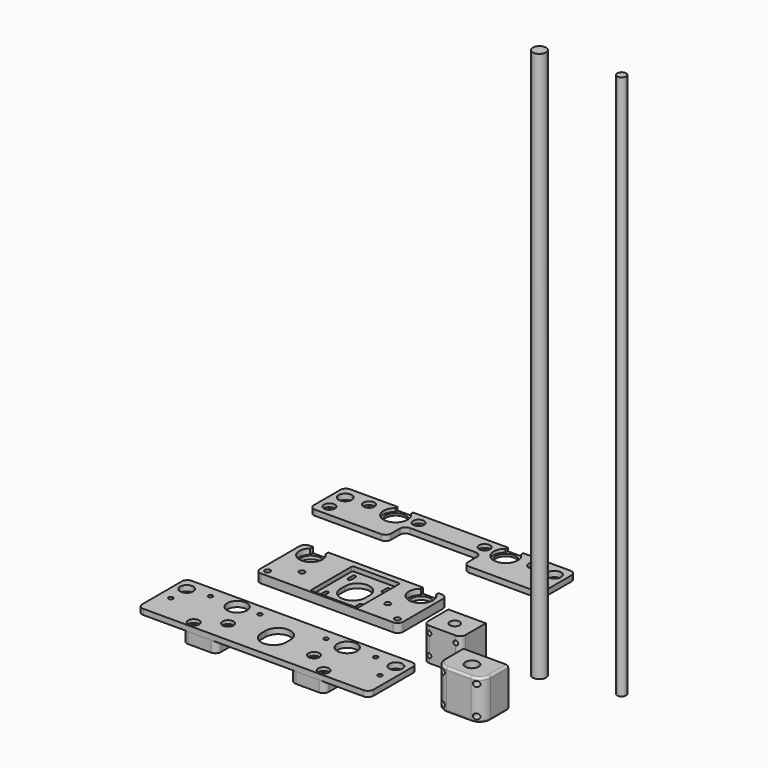
from build123d import *

# Parameters (mm, degrees)
F0_R         = 6
F1_DEPTH     = 500
F2_W         = 130
F2_H         = 55
F2_R         = 2.5
F2_W_2       = 43
F2_H_2       = 48
F2_R_2       = 9
F3_DEPTH     = 8
F4_DEPTH     = 4
F5_R         = 1
F6_R         = 9
F7_DEPTH     = 5
F8_R         = 5
F9_W         = 210
F9_H         = 55
F9_R         = 2.5
F9_R_2       = 2
F9_R_3       = 6
F9_R_4       = 9
F10_DEPTH    = 5
F11_R        = 5
F11_R_2      = 2.5
F12_DEPTH    = 3
F13_R        = 5
F14_W        = 31
F14_H        = 25
F14_R        = 2.5
F15_DEPTH    = 10
F16_R        = 5
F16_2_R      = 5
F17_R        = 2
F17_R_2      = 6
F17_R_3      = 9
F18_DEPTH    = 5
F19_R        = 9
F19_R_2      = 5
F19_R_3      = 2
F20_DEPTH    = 3
F21_R        = 5
F22_W        = 42
F22_H        = 30
F22_R        = 6
F23_DEPTH    = 36
F24_R        = 10
F25_R        = 2
F26_R        = 2.5
F27_DEPTH    = 40
F28_R        = 4
F29_DEPTH    = 495
F30_W        = 34
F30_H        = 28
F30_R        = 4.5
F31_DEPTH    = 30
F32_R        = 2
F33_DEPTH    = 35
F34_T1_DEPTH = 55


# Not quite as in the source:
# - a fillet or chamfer that OpenCascade refuses, or shapes differently, is made with other operations: its cross-section is extruded or revolved along the edge and cut away or added
# - a feature names something its author has since deleted; it is built from what else it names


with BuildPart() as f1:
    # F0 (on Top) → F1 (new body)
    with BuildSketch(Plane.XY):
        with Locations((45.0636185706, 37.0731987059)):
            Circle(F0_R)
    extrude(amount=F1_DEPTH)


with BuildPart() as f3:
    # F2 (on Top) → F3 (new body)
    with BuildSketch(Plane.XY):
        with Locations((-137.1023366213, 51.400513723)):
            Rectangle(F2_W, F2_H)
        with Locations((-196.1023366213, 29.900513723)):
            Circle(F2_R, mode=Mode.SUBTRACT)
        with Locations((-176.1023366213, 43.900513723)):
            Circle(F2_R, mode=Mode.SUBTRACT)
        with Locations((-78.1023366213, 29.900513723)):
            Circle(F2_R, mode=Mode.SUBTRACT)
        with Locations((-132.1023366213, 49.400513723)):
            Rectangle(F2_W_2, F2_H_2, mode=Mode.SUBTRACT)
        with Locations((-98.1023366213, 43.900513723)):
            Circle(F2_R, mode=Mode.SUBTRACT)
        with Locations((-187.1023366213, 67.900513723)):
            Circle(F2_R_2, mode=Mode.SUBTRACT)
        with Locations((-87.1023366213, 67.900513723)):
            Circle(F2_R_2, mode=Mode.SUBTRACT)
    extrude(amount=F3_DEPTH)

    # F2 (on Top) → F4 (join)
    with BuildSketch(Plane.XY):
        with Locations((-132.1023366213, 49.400513723)):
            Rectangle(F2_W_2, F2_H_2)
        with BuildLine():
            Line((-149.1523366213, 31.400513723), (-149.1523366213, 36.400513723))
            ThreePointArc((-149.1523366213, 36.400513723), (-147.6023366213, 37.950513723), (-146.0523366213, 36.400513723))
            Line((-146.0523366213, 36.400513723), (-146.0523366213, 31.400513723))
            ThreePointArc((-146.0523366213, 31.400513723), (-147.6023366213, 29.850513723), (-149.1523366213, 31.400513723))
        make_face(mode=Mode.SUBTRACT)
        with BuildLine():
            Line((-118.1523366213, 31.400513723), (-118.1523366213, 36.400513723))
            ThreePointArc((-118.1523366213, 36.400513723), (-116.6023366213, 37.950513723), (-115.0523366213, 36.400513723))
            Line((-115.0523366213, 36.400513723), (-115.0523366213, 31.400513723))
            ThreePointArc((-115.0523366213, 31.400513723), (-116.6023366213, 29.850513723), (-118.1523366213, 31.400513723))
        make_face(mode=Mode.SUBTRACT)
        with BuildLine():
            Line((-143.3523366213, 46.900513723), (-143.3523366213, 51.900513723))
            ThreePointArc((-143.3523366213, 51.900513723), (-132.1023366213, 63.150513723), (-120.8523366213, 51.900513723))
            Line((-120.8523366213, 51.900513723), (-120.8523366213, 46.900513723))
            ThreePointArc((-120.8523366213, 46.900513723), (-132.1023366213, 35.650513723), (-143.3523366213, 46.900513723))
        make_face(mode=Mode.SUBTRACT)
        with BuildLine():
            Line((-149.1523366213, 62.400513723), (-149.1523366213, 67.400513723))
            ThreePointArc((-149.1523366213, 67.400513723), (-147.6023366213, 68.950513723), (-146.0523366213, 67.400513723))
            Line((-146.0523366213, 67.400513723), (-146.0523366213, 62.400513723))
            ThreePointArc((-146.0523366213, 62.400513723), (-147.6023366213, 60.850513723), (-149.1523366213, 62.400513723))
        make_face(mode=Mode.SUBTRACT)
        with BuildLine():
            Line((-118.1523366213, 62.400513723), (-118.1523366213, 67.400513723))
            ThreePointArc((-118.1523366213, 67.400513723), (-116.6023366213, 68.950513723), (-115.0523366213, 67.400513723))
            Line((-115.0523366213, 67.400513723), (-115.0523366213, 62.400513723))
            ThreePointArc((-115.0523366213, 62.400513723), (-116.6023366213, 60.850513723), (-118.1523366213, 62.400513723))
        make_face(mode=Mode.SUBTRACT)
    extrude(amount=F4_DEPTH)

    # F5
    f5_edges = [f3.edges().sort_by_distance(p)[0] for p in [
        (-153.602337, 73.400514, 6),
        (-110.602337, 73.400514, 6),
        (-110.602337, 25.400514, 6),
        (-153.602337, 25.400514, 6),
    ]]
    fillet(f5_edges, radius=F5_R)

    # F6 (on face) → F7 (cut)
    with BuildSketch(Plane.XY.offset(8)):
        with BuildLine():
            ThreePointArc((-194.1023366213, 75.7267516443), (-191.3889436712, 58.3153689667), (-176.6023366213, 67.900513723))
            ThreePointArc((-176.6023366213, 67.900513723), (-177.5171918649, 72.1871207729), (-180.1023366213, 75.7267516443))
            ThreePointArc((-180.1023366213, 75.7267516443), (-187.1023366213, 78.400513723), (-194.1023366213, 75.7267516443))
        make_face()
        with Locations((-187.1023366213, 67.900513723)):
            Circle(F6_R, mode=Mode.SUBTRACT)
        with BuildLine():
            ThreePointArc((-194.1023366213, 75.7267516443), (-187.1023366213, 78.400513723), (-180.1023366213, 75.7267516443))
            Line((-180.1023366213, 75.7267516443), (-180.1023366213, 78.900513723))
            Line((-180.1023366213, 78.900513723), (-194.1023366213, 78.900513723))
            Line((-194.1023366213, 78.900513723), (-194.1023366213, 75.7267516443))
        make_face()
        with BuildLine():
            ThreePointArc((-87.1023366213, 78.900513723), (-90.8213354707, 78.2527621531), (-94.1023366213, 76.3857950973))
            ThreePointArc((-94.1023366213, 76.3857950973), (-91.7927523811, 57.950639352), (-76.1023366213, 67.900513723))
            ThreePointArc((-76.1023366213, 67.900513723), (-77.1524622502, 72.5909294829), (-80.1023366213, 76.3857950973))
            ThreePointArc((-80.1023366213, 76.3857950973), (-83.3833377719, 78.2527621531), (-87.1023366213, 78.900513723))
        make_face()
        with Locations((-87.1023366213, 67.900513723)):
            Circle(F6_R, mode=Mode.SUBTRACT)
        with BuildLine():
            Line((-87.1023366213, 78.900513723), (-94.1023366213, 78.900513723))
            Line((-94.1023366213, 78.900513723), (-94.1023366213, 76.3857950973))
            ThreePointArc((-94.1023366213, 76.3857950973), (-90.8213354707, 78.2527621531), (-87.1023366213, 78.900513723))
        make_face()
        with BuildLine():
            Line((-80.1023366213, 78.900513723), (-87.1023366213, 78.900513723))
            ThreePointArc((-87.1023366213, 78.900513723), (-83.3833377719, 78.2527621531), (-80.1023366213, 76.3857950973))
            Line((-80.1023366213, 76.3857950973), (-80.1023366213, 78.900513723))
        make_face()
    extrude(amount=-F7_DEPTH, mode=Mode.SUBTRACT)

    # F8
    f8_edges = [f3.edges().sort_by_distance(p)[0] for p in [
        (-202.102337, 78.900514, 4),
        (-202.102337, 23.900514, 4),
        (-72.102337, 23.900514, 4),
        (-72.102337, 78.900514, 4),
    ]]
    fillet(f8_edges, radius=F8_R)


with BuildPart() as f10:
    # F9 (on Top) → F10 (new body)
    with BuildSketch(Plane.XY):
        with Locations((-132.1023366213, -38.599486277)):
            Rectangle(F9_W, F9_H)
        with Locations((-191.1023366213, -60.099486277)):
            Circle(F9_R, mode=Mode.SUBTRACT)
        with Locations((-227.1023366213, -41.099486277)):
            Circle(F9_R_2, mode=Mode.SUBTRACT)
        with Locations((-171.1023366213, -46.099486277)):
            Circle(F9_R, mode=Mode.SUBTRACT)
        with Locations((-73.1023366213, -60.099486277)):
            Circle(F9_R, mode=Mode.SUBTRACT)
        with Locations((-93.1023366213, -46.099486277)):
            Circle(F9_R, mode=Mode.SUBTRACT)
        with BuildLine():
            Line((-143.3523366213, -43.099486277), (-143.3523366213, -38.099486277))
            ThreePointArc((-143.3523366213, -38.099486277), (-132.1023366213, -26.849486277), (-120.8523366213, -38.099486277))
            Line((-120.8523366213, -38.099486277), (-120.8523366213, -43.099486277))
            ThreePointArc((-120.8523366213, -43.099486277), (-132.1023366213, -54.349486277), (-143.3523366213, -43.099486277))
        make_face(mode=Mode.SUBTRACT)
        with Locations((-37.1023366213, -41.099486277)):
            Circle(F9_R_2, mode=Mode.SUBTRACT)
        with Locations((-227.1023366213, -23.099486277)):
            Circle(F9_R_3, mode=Mode.SUBTRACT)
        with Locations((-207.1023366213, -21.099486277)):
            Circle(F9_R_2, mode=Mode.SUBTRACT)
        with Locations((-182.1023366213, -22.099486277)):
            Circle(F9_R_4, mode=Mode.SUBTRACT)
        with Locations((-162.1023366213, -21.099486277)):
            Circle(F9_R_2, mode=Mode.SUBTRACT)
        with Locations((-82.1023366213, -22.099486277)):
            Circle(F9_R_4, mode=Mode.SUBTRACT)
        with Locations((-102.1023366213, -21.099486277)):
            Circle(F9_R_2, mode=Mode.SUBTRACT)
        with Locations((-57.1023366213, -21.099486277)):
            Circle(F9_R_2, mode=Mode.SUBTRACT)
        with Locations((-37.1023366213, -23.099486277)):
            Circle(F9_R_3, mode=Mode.SUBTRACT)
    extrude(amount=F10_DEPTH)

    # F11 (on face) → F12 (cut)
    with BuildSketch(Plane.XY.offset(5)):
        with Locations((-191.1023366213, -60.099486277)):
            Circle(F11_R)
        with Locations((-191.1023366213, -60.099486277)):
            Circle(F11_R_2, mode=Mode.SUBTRACT)
        with Locations((-171.1023366213, -46.099486277)):
            Circle(F11_R)
        with Locations((-171.1023366213, -46.099486277)):
            Circle(F11_R_2, mode=Mode.SUBTRACT)
        with Locations((-93.1023366213, -46.099486277)):
            Circle(F11_R)
        with Locations((-93.1023366213, -46.099486277)):
            Circle(F11_R_2, mode=Mode.SUBTRACT)
        with Locations((-73.1023366213, -60.099486277)):
            Circle(F11_R)
        with Locations((-73.1023366213, -60.099486277)):
            Circle(F11_R_2, mode=Mode.SUBTRACT)
    extrude(amount=-F12_DEPTH, mode=Mode.SUBTRACT)

    # F13
    f13_edges = [f10.edges().sort_by_distance(p)[0] for p in [
        (-237.102337, -11.099486, 2.5),
        (-237.102337, -66.099486, 2.5),
        (-27.102337, -66.099486, 2.5),
        (-27.102337, -11.099486, 2.5),
    ]]
    fillet(f13_edges, radius=F13_R)


with BuildPart() as f15:
    # F14 (on face) → F15 (new body)
    with BuildSketch(Plane(origin=(0, 0, 0), x_dir=(1, 0, 0), z_dir=(0, 0, -1))):
        with Locations((-83.1023366213, 53.599486277)):
            Rectangle(F14_W, F14_H)
        with Locations((-93.1023366213, 46.099486277)):
            Circle(F14_R, mode=Mode.SUBTRACT)
        with Locations((-73.1023366213, 60.099486277)):
            Circle(F14_R, mode=Mode.SUBTRACT)
    extrude(amount=F15_DEPTH)

    # F16
    f16_edges = [f15.edges().sort_by_distance(p)[0] for p in [
        (-98.602337, -66.099486, -5),
        (-98.602337, -41.099486, -5),
        (-67.602337, -66.099486, -5),
        (-67.602337, -41.099486, -5),
    ]]
    fillet(f16_edges, radius=F16_R)


with BuildPart() as f15b:
    # F14 (on face) → F15, piece 2 (new body)
    with BuildSketch(Plane(origin=(0, 0, 0), x_dir=(1, 0, 0), z_dir=(0, 0, -1))):
        with Locations((-181.1023366213, 53.599486277)):
            Rectangle(F14_W, F14_H)
        with Locations((-171.1023366213, 46.099486277)):
            Circle(F14_R, mode=Mode.SUBTRACT)
        with Locations((-191.1023366213, 60.099486277)):
            Circle(F14_R, mode=Mode.SUBTRACT)
    extrude(amount=F15_DEPTH)

    # F16#2
    f16_2_edges = [f15b.edges().sort_by_distance(p)[0] for p in [
        (-165.602337, -41.099486, -5),
        (-165.602337, -66.099486, -5),
        (-196.602337, -66.099486, -5),
        (-196.602337, -41.099486, -5),
    ]]
    fillet(f16_2_edges, radius=F16_2_R)


with BuildPart() as f18:
    # F17 (on Top) → F18 (new body)
    with BuildSketch(Plane.XY):
        Polygon((-27.1023366213, 168.900513723), (-237.1023366213, 168.900513723), (-237.1023366213, 128.900513723), (-167.1023366213, 128.900513723), (-167.1023366213, 148.900513723), (-97.1023366213, 148.900513723), (-97.1023366213, 128.900513723), (-27.1023366213, 128.900513723), align=None)
        with Locations((-227.1023366213, 138.900513723)):
            Circle(F17_R, mode=Mode.SUBTRACT)
        with Locations((-37.1023366213, 138.900513723)):
            Circle(F17_R, mode=Mode.SUBTRACT)
        with Locations((-227.1023366213, 156.900513723)):
            Circle(F17_R_2, mode=Mode.SUBTRACT)
        with Locations((-207.1023366213, 158.900513723)):
            Circle(F17_R, mode=Mode.SUBTRACT)
        with Locations((-182.1023366213, 157.900513723)):
            Circle(F17_R_3, mode=Mode.SUBTRACT)
        with Locations((-162.1023366213, 158.900513723)):
            Circle(F17_R, mode=Mode.SUBTRACT)
        with Locations((-102.1023366213, 158.900513723)):
            Circle(F17_R, mode=Mode.SUBTRACT)
        with Locations((-82.1023366213, 157.900513723)):
            Circle(F17_R_3, mode=Mode.SUBTRACT)
        with Locations((-57.1023366213, 158.900513723)):
            Circle(F17_R, mode=Mode.SUBTRACT)
        with Locations((-37.1023366213, 156.900513723)):
            Circle(F17_R_2, mode=Mode.SUBTRACT)
    extrude(amount=F18_DEPTH)

    # F19 (on face) → F20 (cut)
    with BuildSketch(Plane.XY.offset(5)):
        with BuildLine():
            ThreePointArc((-82.1023366213, 168.900513723), (-85.8213354707, 168.2527621531), (-89.1023366213, 166.3857950973))
            ThreePointArc((-89.1023366213, 166.3857950973), (-86.7927523811, 147.950639352), (-71.1023366213, 157.900513723))
            ThreePointArc((-71.1023366213, 157.900513723), (-72.1524622502, 162.5909294829), (-75.1023366213, 166.3857950973))
            ThreePointArc((-75.1023366213, 166.3857950973), (-78.3833377719, 168.2527621531), (-82.1023366213, 168.900513723))
        make_face()
        with Locations((-82.1023366213, 157.900513723)):
            Circle(F19_R, mode=Mode.SUBTRACT)
        with Locations((-102.1023366213, 158.900513723)):
            Circle(F19_R_2)
        with Locations((-102.1023366213, 158.900513723)):
            Circle(F19_R_3, mode=Mode.SUBTRACT)
        with Locations((-57.1023366213, 158.900513723)):
            Circle(F19_R_2)
        with Locations((-57.1023366213, 158.900513723)):
            Circle(F19_R_3, mode=Mode.SUBTRACT)
        with Locations((-37.1023366213, 138.900513723)):
            Circle(F19_R_2)
        with Locations((-37.1023366213, 138.900513723)):
            Circle(F19_R_3, mode=Mode.SUBTRACT)
        with Locations((-162.1023366213, 158.900513723)):
            Circle(F19_R_2)
        with Locations((-162.1023366213, 158.900513723)):
            Circle(F19_R_3, mode=Mode.SUBTRACT)
        with BuildLine():
            ThreePointArc((-189.1023366213, 166.3857950973), (-186.7927523811, 147.950639352), (-171.1023366213, 157.900513723))
            ThreePointArc((-171.1023366213, 157.900513723), (-172.1524622502, 162.5909294829), (-175.1023366213, 166.3857950973))
            ThreePointArc((-175.1023366213, 166.3857950973), (-178.3833377719, 168.2527621531), (-182.1023366213, 168.900513723))
            ThreePointArc((-182.1023366213, 168.900513723), (-185.8213354707, 168.2527621531), (-189.1023366213, 166.3857950973))
        make_face()
        with Locations((-182.1023366213, 157.900513723)):
            Circle(F19_R, mode=Mode.SUBTRACT)
        with Locations((-207.1023366213, 158.900513723)):
            Circle(F19_R_2)
        with Locations((-207.1023366213, 158.900513723)):
            Circle(F19_R_3, mode=Mode.SUBTRACT)
        with Locations((-227.1023366213, 138.900513723)):
            Circle(F19_R_2)
        with Locations((-227.1023366213, 138.900513723)):
            Circle(F19_R_3, mode=Mode.SUBTRACT)
        with BuildLine():
            Line((-189.1023366213, 168.900513723), (-189.1023366213, 166.3857950973))
            ThreePointArc((-189.1023366213, 166.3857950973), (-185.8213354707, 168.2527621531), (-182.1023366213, 168.900513723))
            Line((-182.1023366213, 168.900513723), (-189.1023366213, 168.900513723))
        make_face()
        with BuildLine():
            ThreePointArc((-182.1023366213, 168.900513723), (-178.3833377719, 168.2527621531), (-175.1023366213, 166.3857950973))
            Line((-175.1023366213, 166.3857950973), (-175.1023366213, 168.900513723))
            Line((-175.1023366213, 168.900513723), (-182.1023366213, 168.900513723))
        make_face()
        with BuildLine():
            Line((-82.1023366213, 168.900513723), (-89.1023366213, 168.900513723))
            Line((-89.1023366213, 168.900513723), (-89.1023366213, 166.3857950973))
            ThreePointArc((-89.1023366213, 166.3857950973), (-85.8213354707, 168.2527621531), (-82.1023366213, 168.900513723))
        make_face()
        with BuildLine():
            Line((-75.1023366213, 168.900513723), (-82.1023366213, 168.900513723))
            ThreePointArc((-82.1023366213, 168.900513723), (-78.3833377719, 168.2527621531), (-75.1023366213, 166.3857950973))
            Line((-75.1023366213, 166.3857950973), (-75.1023366213, 168.900513723))
        make_face()
    extrude(amount=-F20_DEPTH, mode=Mode.SUBTRACT)

    # F21
    f21_edges = [f18.edges().sort_by_distance(p)[0] for p in [
        (-237.102337, 128.900514, 2.5),
        (-237.102337, 168.900514, 2.5),
        (-167.102337, 128.900514, 2.5),
        (-167.102337, 148.900514, 2.5),
        (-97.102337, 148.900514, 2.5),
        (-97.102337, 128.900514, 2.5),
        (-27.102337, 128.900514, 2.5),
        (-27.102337, 168.900514, 2.5),
    ]]
    fillet(f21_edges, radius=F21_R)


with BuildPart() as f23:
    # F22 (on Top) → F23 (new body)
    with BuildSketch(Plane.XY):
        with Locations((40.410891258, -33.6393057252)):
            Rectangle(F22_W, F22_H)
        with Locations((40.410891258, -33.6393057252)):
            Circle(F22_R, mode=Mode.SUBTRACT)
    extrude(amount=F23_DEPTH)

    # F24
    f24_edges = [f23.edges().sort_by_distance(p)[0] for p in [
        (19.410891, -48.639306, 18),
        (61.410891, -48.639306, 18),
    ]]
    fillet(f24_edges, radius=F24_R)

    # F25
    f25_edges = [f23.edges().sort_by_distance(p)[0] for p in [
        (40.410891, -48.639306, 36),
        (61.410891, -28.639306, 0),
    ]]
    fillet(f25_edges, radius=F25_R)

    # F26 (on face) → F27 (cut)
    with BuildSketch(Plane(origin=(0, -18.6393057252, 0), x_dir=(-1, 0, 0), z_dir=(0, 1, 0))):
        with Locations((-25.160891258, 5)):
            Circle(F26_R)
        with Locations((-25.160891258, 31)):
            Circle(F26_R)
        with Locations((-55.660891258, 31)):
            Circle(F26_R)
        with Locations((-55.660891258, 5)):
            Circle(F26_R)
    extrude(amount=-F27_DEPTH, mode=Mode.SUBTRACT)


with BuildPart() as f29:
    # F28 (on Top) → F29 (new body)
    with BuildSketch(Plane.XY):
        with Locations((108.4851548076, 51.2675791979)):
            Circle(F28_R)
    extrude(amount=F29_DEPTH)


with BuildPart() as f31:
    # F30 (on Top) → F31 (new body)
    with BuildSketch(Plane.XY):
        with Locations((-15.5411828693, 16.8240186758)):
            Rectangle(F30_W, F30_H)
        with Locations((-15.5411828693, 16.8240186758)):
            Circle(F30_R, mode=Mode.SUBTRACT)
    extrude(amount=F31_DEPTH)

    # F32 (on face) → F33 (cut)
    with BuildSketch(Plane(origin=(0, 30.8240186758, 0), x_dir=(-1, 0, 0), z_dir=(0, 1, 0))):
        with Locations((27.5411828693, 24)):
            Circle(F32_R)
        with Locations((3.5411828693, 24)):
            Circle(F32_R)
        with Locations((3.5411828693, 6)):
            Circle(F32_R)
        with Locations((27.5411828693, 6)):
            Circle(F32_R)
    extrude(amount=-F33_DEPTH, mode=Mode.SUBTRACT)

    # F34: fillet of radius 5 on 2 edges, made by hand

    # F34_s2 → F34_t1 (cut)
    with BuildSketch(Plane.XY.offset(-12.5)):
        with BuildLine():
            ThreePointArc((-27.5411828693, 2.8240186758), (-31.0767167752, 4.2884847699), (-32.5411828693, 7.8240186758))
            Line((-32.5411828693, 7.8240186758), (-32.5411828693, 2.8240186758))
            Line((-32.5411828693, 2.8240186758), (-27.5411828693, 2.8240186758))
        make_face()
        with BuildLine():
            ThreePointArc((1.4588171307, 7.8240186758), (-0.0056489634, 4.2884847699), (-3.5411828693, 2.8240186758))
            Line((-3.5411828693, 2.8240186758), (1.4588171307, 2.8240186758))
            Line((1.4588171307, 2.8240186758), (1.4588171307, 7.8240186758))
        make_face()
    extrude(amount=F34_T1_DEPTH, mode=Mode.SUBTRACT)


solid = Compound([f1.part, f3.part, f10.part, f15.part, f15b.part, f18.part, f23.part, f29.part, f31.part])
